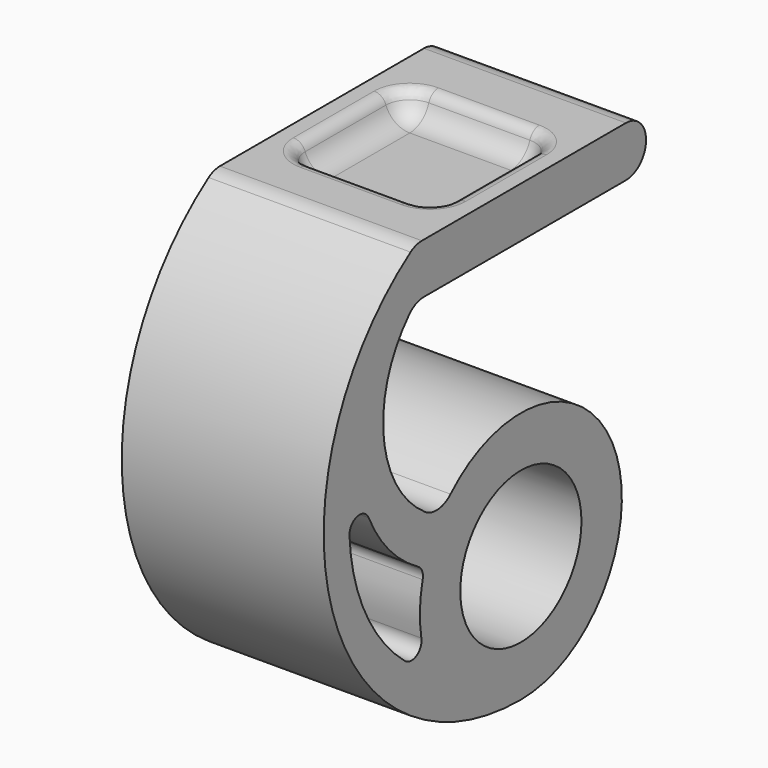
from build123d import *

# Parameters (mm, degrees)
F0_R         = 9.525
F1_DEPTH     = 25.4
F2_W         = 19.05
F2_H         = 19.05
F3_DEPTH     = 3.175
F4_T1_DEPTH  = 25.4
F4_T3_DEPTH  = 12.7
F4_T5_DEPTH  = 12.7
F4_S9_W      = 3.175
F4_S9_H      = 3.175
F4_T10_DEPTH = 3.175
F4_S15_W     = 3.175
F4_S15_H     = 3.175
F4_T16_DEPTH = 3.175
F4_S21_W     = 3.175
F4_S21_H     = 3.175
F4_T22_DEPTH = 3.175
F4_S27_W     = 3.175
F4_S27_H     = 3.175
F4_T28_DEPTH = 3.175
F4_T31_DEPTH = 30.3662191739
F5_R         = 1.5875


# Not quite as in the source:
# - a fillet or chamfer that OpenCascade refuses, or shapes differently, is made with other operations: its cross-section is extruded or revolved along the edge and cut away or added


with BuildPart() as f1:
    # F0 (on Right) → F1 (new body)
    with BuildSketch(Plane.YZ):
        with BuildLine():
            Line((16.51, 15.875), (-16.51, 15.875))
            ThreePointArc((-16.51, 15.875), (-29.7854143214, -18.9198974706), (0, -41.275))
            ThreePointArc((0, -41.275), (14.2378547718, -18.3786670428), (-12.5944842771, -15.7359123145))
            ThreePointArc((-12.5944842771, -15.7359123145), (-21.4720341133, -4.1780442704), (-16.51, 9.525))
            Line((-16.51, 9.525), (16.51, 9.525))
            ThreePointArc((16.51, 9.525), (19.685, 12.7), (16.51, 15.875))
        make_face()
        with BuildLine():
            ThreePointArc((-14.343097751, -32.2037615996), (-25.3220142156, -19.7737801421), (-25.6780404598, -3.1932406127))
            ThreePointArc((-25.6780404598, -3.1932406127), (-22.8730710881, -13.3775496244), (-15.115016679, -20.5469704521))
            ThreePointArc((-15.115016679, -20.5469704521), (-15.8403068596, -26.4489535701), (-14.343097751, -32.2037615996))
        make_face(mode=Mode.SUBTRACT)
        with Locations((0, -25.4)):
            Circle(F0_R, mode=Mode.SUBTRACT)
    extrude(amount=F1_DEPTH)

    # F2 (on face) → F3 (cut)
    with BuildSketch(Plane.XY.offset(15.875)):
        with Locations((12.7, 0)):
            Rectangle(F2_W, F2_H)
    extrude(amount=-F3_DEPTH, mode=Mode.SUBTRACT)

    # F4: fillet of radius 3.175 on 11 edges, made by hand

    # F4_s2 → F4_t1 (join)
    with BuildSketch(Plane.YZ):
        with BuildLine():
            ThreePointArc((-15.229163377, 9.525), (-16.4906498384, 9.2636363719), (-17.5444470536, 8.5225760049))
            ThreePointArc((-17.5444470536, 8.5225760049), (-17.0391316289, 9.0360765162), (-16.51, 9.525))
            Line((-16.51, 9.525), (-15.229163377, 9.525))
        make_face()
        with BuildLine():
            ThreePointArc((-15.0737959989, -14.3545542957), (-13.0077413525, -14.9014210416), (-11.0631237972, -14.0147939479))
            ThreePointArc((-11.0631237972, -14.0147939479), (-11.8600660646, -14.8475378256), (-12.5944842771, -15.7359123145))
            ThreePointArc((-12.5944842771, -15.7359123145), (-13.8665248674, -15.1033585978), (-15.0737959989, -14.3545542957))
        make_face()
    extrude(amount=F4_T1_DEPTH)

    # F4_s4 → F4_t3 (join)
    with BuildSketch(Plane.YZ.offset(6.35)):
        with BuildLine():
            ThreePointArc((9.525, 15.875), (8.5950640303, 13.6299359697), (6.35, 12.7))
            Line((6.35, 12.7), (9.525, 12.7))
            Line((9.525, 12.7), (9.525, 15.875))
        make_face()
        with BuildLine():
            ThreePointArc((-9.525, 15.875), (-8.5950640303, 13.6299359697), (-6.35, 12.7))
            Line((-6.35, 12.7), (-9.525, 12.7))
            Line((-9.525, 12.7), (-9.525, 15.875))
        make_face()
    extrude(amount=F4_T3_DEPTH)

    # F4_s6 → F4_t5 (join)
    with BuildSketch(Plane.XZ.offset(-6.35)):
        with BuildLine():
            ThreePointArc((3.175, 15.875), (4.1049359697, 13.6299359697), (6.35, 12.7))
            Line((6.35, 12.7), (3.175, 12.7))
            Line((3.175, 12.7), (3.175, 15.875))
        make_face()
        with BuildLine():
            ThreePointArc((22.225, 15.875), (21.2950640303, 13.6299359697), (19.05, 12.7))
            Line((19.05, 12.7), (22.225, 12.7))
            Line((22.225, 12.7), (22.225, 15.875))
        make_face()
    extrude(amount=F4_T5_DEPTH)


with BuildPart() as f4_tool8:
    # F4_s9 → F4_t10 (new body)
    with BuildSketch(Plane.XY.offset(15.875)):
        with Locations((20.6375, 7.9375)):
            Rectangle(F4_S9_W, F4_S9_H)
    extrude(amount=-F4_T10_DEPTH)

    # F4_s11 → F4_t12 (revolve, cut)
    with BuildSketch(Plane(origin=(19.05, 6.35, 15.875), x_dir=(-0.7071067812, -0.7071067812, 0), z_dir=(0.7071067812, -0.7071067812, 0))):
        with BuildLine():
            ThreePointArc((0, -3.175), (3.175, 0), (0, 3.175))
            Line((0, 3.175), (0, -3.175))
        make_face()
    revolve(axis=Axis((19.05, 6.35, 15.875), (0, 0, -1)), mode=Mode.SUBTRACT)


with BuildPart() as f1_1:
    add(f1.part)

    # F4_t7: union F4_tool8
    add(f4_tool8.part)


with BuildPart() as f4_tool14:
    # F4_s15 → F4_t16 (new body)
    with BuildSketch(Plane.XY.offset(15.875)):
        with Locations((4.7625, 7.9375)):
            Rectangle(F4_S15_W, F4_S15_H)
    extrude(amount=-F4_T16_DEPTH)

    # F4_s17 → F4_t18 (revolve, cut)
    with BuildSketch(Plane(origin=(6.35, 6.35, 15.875), x_dir=(0.7071067812, -0.7071067812, 0), z_dir=(0.7071067812, 0.7071067812, 0))):
        with BuildLine():
            ThreePointArc((0, -3.175), (3.175, 0), (0, 3.175))
            Line((0, 3.175), (0, -3.175))
        make_face()
    revolve(axis=Axis((6.35, 6.35, 15.875), (0, 0, -1)), mode=Mode.SUBTRACT)


with BuildPart() as f1_2:
    add(f1_1.part)

    # F4_t13: union F4_tool14
    add(f4_tool14.part)


with BuildPart() as f4_tool20:
    # F4_s21 → F4_t22 (new body)
    with BuildSketch(Plane.XY.offset(15.875)):
        with Locations((4.7625, -7.9375)):
            Rectangle(F4_S21_W, F4_S21_H)
    extrude(amount=-F4_T22_DEPTH)

    # F4_s23 → F4_t24 (revolve, cut)
    with BuildSketch(Plane(origin=(6.35, -6.35, 15.875), x_dir=(0.7071067812, 0.7071067812, 0), z_dir=(-0.7071067812, 0.7071067812, 0))):
        with BuildLine():
            ThreePointArc((0, -3.175), (3.175, 0), (0, 3.175))
            Line((0, 3.175), (0, -3.175))
        make_face()
    revolve(axis=Axis((6.35, -6.35, 15.875), (0, 0, -1)), mode=Mode.SUBTRACT)


with BuildPart() as f1_3:
    add(f1_2.part)

    # F4_t19: union F4_tool20
    add(f4_tool20.part)


with BuildPart() as f4_tool26:
    # F4_s27 → F4_t28 (new body)
    with BuildSketch(Plane.XY.offset(15.875)):
        with Locations((20.6375, -7.9375)):
            Rectangle(F4_S27_W, F4_S27_H)
    extrude(amount=-F4_T28_DEPTH)

    # F4_s29 → F4_t30 (revolve, cut)
    with BuildSketch(Plane(origin=(19.05, -6.35, 15.875), x_dir=(-0.7071067812, 0.7071067812, 0), z_dir=(-0.7071067812, -0.7071067812, 0))):
        with BuildLine():
            ThreePointArc((0, -3.175), (3.175, 0), (0, 3.175))
            Line((0, 3.175), (0, -3.175))
        make_face()
    revolve(axis=Axis((19.05, -6.35, 15.875), (0, 0, -1)), mode=Mode.SUBTRACT)


with BuildPart() as f1_4:
    add(f1_3.part)

    # F4_t25: union F4_tool26
    add(f4_tool26.part)

    # F4_s32 → F4_t31 (cut)
    with BuildSketch(Plane.YZ.offset(-2.483109587)):
        with BuildLine():
            ThreePointArc((-15.5690922553, 15.875), (-16.4962795763, 15.7366015003), (-17.3426345609, 15.3334716042))
            ThreePointArc((-17.3426345609, 15.3334716042), (-16.9284902387, 15.6075768645), (-16.51, 15.875))
            Line((-16.51, 15.875), (-15.5690922553, 15.875))
        make_face()
    extrude(amount=F4_T31_DEPTH, mode=Mode.SUBTRACT)

    # F5
    f5_edges = [f1_4.edges().sort_by_distance(p)[0] for p in [
        (12.7, -9.525, 15.875),
        (3.175, 0, 15.875),
        (12.7, 9.525, 15.875),
        (22.225, 0, 15.875),
        (12.7, -15.115017, -20.54697),
        (12.7, -14.343098, -32.203762),
        (12.7, -25.67804, -3.193241),
        (21.295064, 8.595064, 15.875),
        (21.295064, -8.595064, 15.875),
        (4.104936, 8.595064, 15.875),
        (4.104936, -8.595064, 15.875),
    ]]
    fillet(f5_edges, radius=F5_R)


solid = f1_4.part
